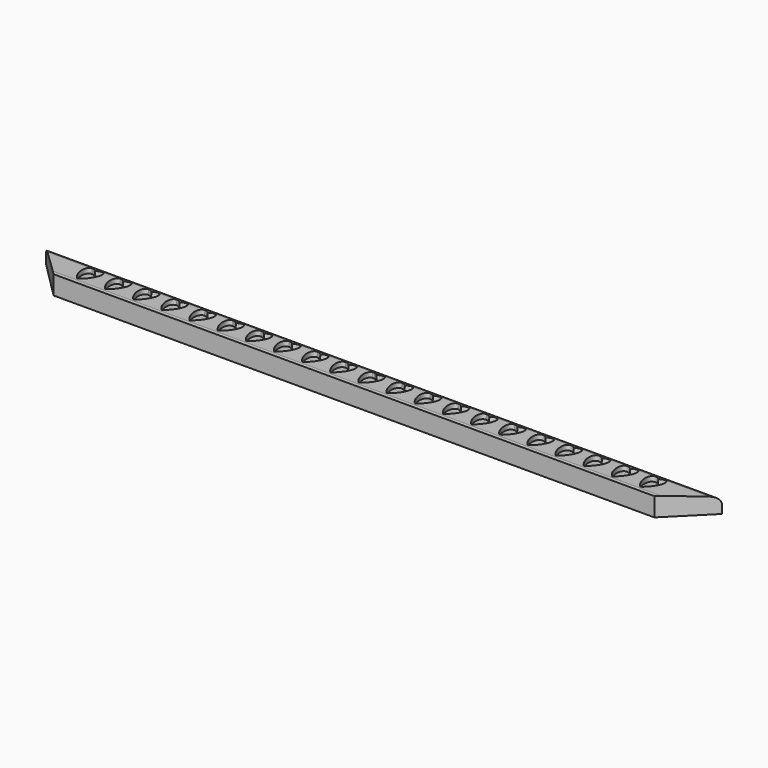
from build123d import *

# Parameters (mm, degrees)
F1_DEPTH = 12.7
F2_SIZE2 = 22.86
F2_SIZE  = 2.54
F3_R     = 5.08
F5_DEPTH = 3.175


# Not quite as in the source:
# - a feature names something its author has since deleted; it is built from what else it names


with BuildPart() as f1:
    # F0 (on Top) → F1 (new body)
    with BuildSketch(Plane.XY):
        Polygon((228.6, 12.7), (-228.6, 12.7), (-203.2, -12.7), (203.2, -12.7), align=None)
    extrude(amount=F1_DEPTH)

    # F2
    f2_edges = [f1.edges().sort_by_distance(p)[0] for p in [
        (0, 12.7, 12.7),
    ]]
    f2_side = f1.faces().sort_by_distance((0, 12.7, 6.35))[0]
    chamfer(f2_edges, length=F2_SIZE, length2=F2_SIZE2, reference=f2_side)

    # F3
    f3_edges = [f1.edges().sort_by_distance(p)[0] for p in [
        (0, 12.7, 10.16),
    ]]
    fillet(f3_edges, radius=F3_R)

    # F4 (on face) → F5 (cut)
    with BuildSketch(Plane(origin=(0, 1.27, 11.43), x_dir=(1, 0, 0), z_dir=(0, 0.1104315261, 0.9938837347))):
        with BuildLine():
            add(Edge.make_bspline(
                [(-190.5, 5.3298376858), (-192.2906218206, 6.9535217541), (-193.7692225246, 6.9535217364)],
                knots=[5.4853328791, 5.4853328791, 5.4853328791, 6.084603808, 6.084603808, 6.084603808], degree=2, weights=[1, 0.9554441533, 1]))
            add(Edge.make_bspline(
                [(-193.7692225246, 6.9535217364), (-209.2613622208, 6.95352155), (-190.5, -10.058738989)],
                knots=[6.084603808, 6.084603808, 6.084603808, 8.6269255327, 8.6269255327, 8.6269255327], degree=2, weights=[1, 0.2951719329, 1]))
            add(Edge.make_bspline(
                [(-190.5, -10.058738989), (-171.7386375737, 6.9535217364), (-187.2307775049, 6.9535217364)],
                knots=[3.9394450816, 3.9394450816, 3.9394450816, 6.4817668125, 6.4817668125, 6.4817668125], degree=2, weights=[1, 0.29517193, 1]))
            add(Edge.make_bspline(
                [(-187.2307775049, 6.9535217364), (-188.709378199, 6.9535217364), (-190.5, 5.3298376858)],
                knots=[0.1985815053, 0.1985815053, 0.1985815053, 0.797852428, 0.797852428, 0.797852428], degree=2, weights=[1, 0.9554441542, 1]))
        make_face()
        with BuildLine():
            add(Edge.make_bspline(
                [(-171.45, 5.3298376858), (-173.2406217996, 6.9535217351), (-174.719222493, 6.9535217364)],
                knots=[5.4853328791, 5.4853328791, 5.4853328791, 6.0846038014, 6.0846038014, 6.0846038014], degree=2, weights=[1, 0.9554441542, 1]))
            add(Edge.make_bspline(
                [(-174.719222493, 6.9535217364), (-190.2113624409, 6.9535217496), (-171.45, -10.058738989)],
                knots=[6.0846038014, 6.0846038014, 6.0846038014, 8.6269255327, 8.6269255327, 8.6269255327], degree=2, weights=[1, 0.2951719298, 1]))
            add(Edge.make_bspline(
                [(-171.45, -10.058738989), (-152.6886375737, 6.9535217364), (-168.1807775049, 6.9535217364)],
                knots=[3.9394450816, 3.9394450816, 3.9394450816, 6.4817668125, 6.4817668125, 6.4817668125], degree=2, weights=[1, 0.29517193, 1]))
            add(Edge.make_bspline(
                [(-168.1807775049, 6.9535217364), (-169.659378199, 6.9535217364), (-171.45, 5.3298376858)],
                knots=[0.1985815053, 0.1985815053, 0.1985815053, 0.797852428, 0.797852428, 0.797852428], degree=2, weights=[1, 0.9554441542, 1]))
        make_face()
        with BuildLine():
            add(Edge.make_bspline(
                [(-152.4, 5.3298376858), (-154.190621801, 6.9535217364), (-155.6692224951, 6.9535217364)],
                knots=[5.4853328791, 5.4853328791, 5.4853328791, 6.0846038019, 6.0846038019, 6.0846038019], degree=2, weights=[1, 0.9554441542, 1]))
            add(Edge.make_bspline(
                [(-155.6692224951, 6.9535217364), (-171.1613624263, 6.9535217363), (-152.4, -10.058738989)],
                knots=[6.0846038019, 6.0846038019, 6.0846038019, 8.6269255327, 8.6269255327, 8.6269255327], degree=2, weights=[1, 0.29517193, 1]))
            add(Edge.make_bspline(
                [(-152.4, -10.058738989), (-133.6386378713, 6.9535214665), (-149.1307774621, 6.9535217364)],
                knots=[3.9394450816, 3.9394450816, 3.9394450816, 6.4817668036, 6.4817668036, 6.4817668036], degree=2, weights=[1, 0.2951719342, 1]))
            add(Edge.make_bspline(
                [(-149.1307774621, 6.9535217364), (-150.6093781706, 6.9535217621), (-152.4, 5.3298376858)],
                knots=[0.1985814964, 0.1985814964, 0.1985814964, 0.797852428, 0.797852428, 0.797852428], degree=2, weights=[1, 0.9554441529, 1]))
        make_face()
        with BuildLine():
            add(Edge.make_bspline(
                [(-133.35, 5.3298376858), (-135.140621801, 6.9535217364), (-136.6192224951, 6.9535217364)],
                knots=[5.4853328791, 5.4853328791, 5.4853328791, 6.0846038019, 6.0846038019, 6.0846038019], degree=2, weights=[1, 0.9554441542, 1]))
            add(Edge.make_bspline(
                [(-136.6192224951, 6.9535217364), (-152.1113624263, 6.9535217363), (-133.35, -10.058738989)],
                knots=[6.0846038019, 6.0846038019, 6.0846038019, 8.6269255327, 8.6269255327, 8.6269255327], degree=2, weights=[1, 0.29517193, 1]))
            add(Edge.make_bspline(
                [(-133.35, -10.058738989), (-114.5886378713, 6.9535214665), (-130.0807774621, 6.9535217364)],
                knots=[3.9394450816, 3.9394450816, 3.9394450816, 6.4817668036, 6.4817668036, 6.4817668036], degree=2, weights=[1, 0.2951719342, 1]))
            add(Edge.make_bspline(
                [(-130.0807774621, 6.9535217364), (-131.5593781706, 6.9535217621), (-133.35, 5.3298376858)],
                knots=[0.1985814964, 0.1985814964, 0.1985814964, 0.797852428, 0.797852428, 0.797852428], degree=2, weights=[1, 0.9554441529, 1]))
        make_face()
        with BuildLine():
            add(Edge.make_bspline(
                [(-114.3, 5.3298376858), (-116.0906217421, 6.953521683), (-117.5692224063, 6.9535217364)],
                knots=[5.4853328791, 5.4853328791, 5.4853328791, 6.0846037833, 6.0846037833, 6.0846037833], degree=2, weights=[1, 0.9554441569, 1]))
            add(Edge.make_bspline(
                [(-117.5692224063, 6.9535217364), (-133.0613630431, 6.9535222957), (-114.3, -10.058738989)],
                knots=[6.0846037833, 6.0846037833, 6.0846037833, 8.6269255327, 8.6269255327, 8.6269255327], degree=2, weights=[1, 0.2951719211, 1]))
            add(Edge.make_bspline(
                [(-114.3, -10.058738989), (-95.5386373164, 6.9535219697), (-111.030777542, 6.9535217364)],
                knots=[3.9394450816, 3.9394450816, 3.9394450816, 6.4817668202, 6.4817668202, 6.4817668202], degree=2, weights=[1, 0.2951719263, 1]))
            add(Edge.make_bspline(
                [(-111.030777542, 6.9535217364), (-112.5093782236, 6.9535217141), (-114.3, 5.3298376858)],
                knots=[0.1985815131, 0.1985815131, 0.1985815131, 0.797852428, 0.797852428, 0.797852428], degree=2, weights=[1, 0.9554441553, 1]))
        make_face()
        with BuildLine():
            add(Edge.make_bspline(
                [(-95.25, -10.058738989), (-76.4886375737, 6.9535217364), (-91.9807775049, 6.9535217364)],
                knots=[3.9394450816, 3.9394450816, 3.9394450816, 6.4817668125, 6.4817668125, 6.4817668125], degree=2, weights=[1, 0.29517193, 1]))
            add(Edge.make_bspline(
                [(-91.9807775049, 6.9535217364), (-93.459378199, 6.9535217364), (-95.25, 5.3298376858)],
                knots=[0.1985815053, 0.1985815053, 0.1985815053, 0.797852428, 0.797852428, 0.797852428], degree=2, weights=[1, 0.9554441542, 1]))
            add(Edge.make_bspline(
                [(-95.25, 5.3298376858), (-97.0406217996, 6.9535217351), (-98.519222493, 6.9535217364)],
                knots=[5.4853328791, 5.4853328791, 5.4853328791, 6.0846038014, 6.0846038014, 6.0846038014], degree=2, weights=[1, 0.9554441542, 1]))
            add(Edge.make_bspline(
                [(-98.519222493, 6.9535217364), (-114.0113624409, 6.9535217496), (-95.25, -10.058738989)],
                knots=[6.0846038014, 6.0846038014, 6.0846038014, 8.6269255327, 8.6269255327, 8.6269255327], degree=2, weights=[1, 0.2951719298, 1]))
        make_face()
        with BuildLine():
            add(Edge.make_bspline(
                [(-76.2, -10.058738989), (-57.438637273, 6.953522009), (-72.9307775482, 6.9535217364)],
                knots=[3.9394450816, 3.9394450816, 3.9394450816, 6.4817668215, 6.4817668215, 6.4817668215], degree=2, weights=[1, 0.2951719256, 1]))
            add(Edge.make_bspline(
                [(-72.9307775482, 6.9535217364), (-74.4093782277, 6.9535217103), (-76.2, 5.3298376858)],
                knots=[0.1985815144, 0.1985815144, 0.1985815144, 0.797852428, 0.797852428, 0.797852428], degree=2, weights=[1, 0.9554441555, 1]))
            add(Edge.make_bspline(
                [(-76.2, 5.3298376858), (-77.9906218599, 6.9535217897), (-79.4692225838, 6.9535217364)],
                knots=[5.4853328791, 5.4853328791, 5.4853328791, 6.0846038204, 6.0846038204, 6.0846038204], degree=2, weights=[1, 0.9554441514, 1]))
            add(Edge.make_bspline(
                [(-79.4692225838, 6.9535217364), (-94.9613618094, 6.953521177), (-76.2, -10.058738989)],
                knots=[6.0846038204, 6.0846038204, 6.0846038204, 8.6269255327, 8.6269255327, 8.6269255327], degree=2, weights=[1, 0.2951719388, 1]))
        make_face()
        with BuildLine():
            add(Edge.make_bspline(
                [(-57.15, -10.058738989), (-38.3886375871, 6.9535217242), (-53.880777503, 6.9535217364)],
                knots=[3.9394450816, 3.9394450816, 3.9394450816, 6.4817668121, 6.4817668121, 6.4817668121], degree=2, weights=[1, 0.2951719302, 1]))
            add(Edge.make_bspline(
                [(-53.880777503, 6.9535217364), (-55.3593781977, 6.9535217375), (-57.15, 5.3298376858)],
                knots=[0.1985815049, 0.1985815049, 0.1985815049, 0.797852428, 0.797852428, 0.797852428], degree=2, weights=[1, 0.9554441541, 1]))
            add(Edge.make_bspline(
                [(-57.15, 5.3298376858), (-58.940621801, 6.9535217364), (-60.4192224951, 6.9535217364)],
                knots=[5.4853328791, 5.4853328791, 5.4853328791, 6.0846038019, 6.0846038019, 6.0846038019], degree=2, weights=[1, 0.9554441542, 1]))
            add(Edge.make_bspline(
                [(-60.4192224951, 6.9535217364), (-75.9113624263, 6.9535217363), (-57.15, -10.058738989)],
                knots=[6.0846038019, 6.0846038019, 6.0846038019, 8.6269255327, 8.6269255327, 8.6269255327], degree=2, weights=[1, 0.29517193, 1]))
        make_face()
        with BuildLine():
            add(Edge.make_bspline(
                [(-38.1, -10.058738989), (-19.3386369435, 6.9535223078), (-34.8307775956, 6.9535217364)],
                knots=[3.9394450816, 3.9394450816, 3.9394450816, 6.4817668315, 6.4817668315, 6.4817668315], degree=2, weights=[1, 0.2951719209, 1]))
            add(Edge.make_bspline(
                [(-34.8307775956, 6.9535217364), (-36.3093782592, 6.9535216818), (-38.1, 5.3298376858)],
                knots=[0.1985815243, 0.1985815243, 0.1985815243, 0.797852428, 0.797852428, 0.797852428], degree=2, weights=[1, 0.955444157, 1]))
            add(Edge.make_bspline(
                [(-38.1, 5.3298376858), (-39.890621801, 6.9535217364), (-41.3692224951, 6.9535217364)],
                knots=[5.4853328791, 5.4853328791, 5.4853328791, 6.0846038019, 6.0846038019, 6.0846038019], degree=2, weights=[1, 0.9554441542, 1]))
            add(Edge.make_bspline(
                [(-41.3692224951, 6.9535217364), (-56.8613624263, 6.9535217363), (-38.1, -10.058738989)],
                knots=[6.0846038019, 6.0846038019, 6.0846038019, 8.6269255327, 8.6269255327, 8.6269255327], degree=2, weights=[1, 0.29517193, 1]))
        make_face()
        with BuildLine():
            add(Edge.make_bspline(
                [(19.05, 5.3298376858), (17.2593782129, 6.9535217237), (15.7807775259, 6.9535217364)],
                knots=[5.4853328791, 5.4853328791, 5.4853328791, 6.0846037975, 6.0846037975, 6.0846037975], degree=2, weights=[1, 0.9554441548, 1]))
            add(Edge.make_bspline(
                [(15.7807775259, 6.9535217364), (0.2886374279, 6.9535218686), (19.05, -10.058738989)],
                knots=[6.0846037975, 6.0846037975, 6.0846037975, 8.6269255327, 8.6269255327, 8.6269255327], degree=2, weights=[1, 0.2951719279, 1]))
            add(Edge.make_bspline(
                [(19.05, -10.058738989), (37.8113620751, 6.9535214179), (22.3192225456, 6.9535217364)],
                knots=[3.9394450816, 3.9394450816, 3.9394450816, 6.4817668019, 6.4817668019, 6.4817668019], degree=2, weights=[1, 0.295171935, 1]))
            add(Edge.make_bspline(
                [(22.3192225456, 6.9535217364), (20.8406218345, 6.9535217667), (19.05, 5.3298376858)],
                knots=[0.1985814948, 0.1985814948, 0.1985814948, 0.797852428, 0.797852428, 0.797852428], degree=2, weights=[1, 0.9554441526, 1]))
        make_face()
        with BuildLine():
            add(Edge.make_bspline(
                [(38.1, 5.3298376858), (36.3093782153, 6.9535217216), (34.8307775295, 6.9535217364)],
                knots=[5.4853328791, 5.4853328791, 5.4853328791, 6.0846037967, 6.0846037967, 6.0846037967], degree=2, weights=[1, 0.9554441549, 1]))
            add(Edge.make_bspline(
                [(34.8307775295, 6.9535217364), (19.3386374032, 6.9535218909), (38.1, -10.058738989)],
                knots=[6.0846037967, 6.0846037967, 6.0846037967, 8.6269255327, 8.6269255327, 8.6269255327], degree=2, weights=[1, 0.2951719275, 1]))
            add(Edge.make_bspline(
                [(38.1, -10.058738989), (56.8613623982, 6.9535217109), (41.3692224991, 6.9535217364)],
                knots=[3.9394450816, 3.9394450816, 3.9394450816, 6.4817668117, 6.4817668117, 6.4817668117], degree=2, weights=[1, 0.2951719304, 1]))
            add(Edge.make_bspline(
                [(41.3692224991, 6.9535217364), (39.8906218037, 6.9535217388), (38.1, 5.3298376858)],
                knots=[0.1985815045, 0.1985815045, 0.1985815045, 0.797852428, 0.797852428, 0.797852428], degree=2, weights=[1, 0.9554441541, 1]))
        make_face()
        with BuildLine():
            add(Edge.make_bspline(
                [(57.15, 5.3298376858), (55.3593781853, 6.9535217488), (53.8807774843, 6.9535217364)],
                knots=[5.4853328791, 5.4853328791, 5.4853328791, 6.0846038062, 6.0846038062, 6.0846038062], degree=2, weights=[1, 0.9554441535, 1]))
            add(Edge.make_bspline(
                [(53.8807774843, 6.9535217364), (38.3886377172, 6.9535216063), (57.15, -10.058738989)],
                knots=[6.0846038062, 6.0846038062, 6.0846038062, 8.6269255327, 8.6269255327, 8.6269255327], degree=2, weights=[1, 0.295171932, 1]))
            add(Edge.make_bspline(
                [(57.15, -10.058738989), (75.9113621555, 6.9535214909), (60.419222534, 6.9535217364)],
                knots=[3.9394450816, 3.9394450816, 3.9394450816, 6.4817668044, 6.4817668044, 6.4817668044], degree=2, weights=[1, 0.2951719339, 1]))
            add(Edge.make_bspline(
                [(60.419222534, 6.9535217364), (58.9406218268, 6.9535217598), (57.15, 5.3298376858)],
                knots=[0.1985814972, 0.1985814972, 0.1985814972, 0.797852428, 0.797852428, 0.797852428], degree=2, weights=[1, 0.955444153, 1]))
        make_face()
        with BuildLine():
            add(Edge.make_bspline(
                [(171.45, -10.058738989), (190.2113625182, 6.9535218197), (174.7192224818, 6.9535217364)],
                knots=[3.9394450816, 3.9394450816, 3.9394450816, 6.4817668153, 6.4817668153, 6.4817668153], degree=2, weights=[1, 0.2951719286, 1]))
            add(Edge.make_bspline(
                [(174.7192224818, 6.9535217364), (173.2406217922, 6.9535217284), (171.45, 5.3298376858)],
                knots=[0.1985815081, 0.1985815081, 0.1985815081, 0.797852428, 0.797852428, 0.797852428], degree=2, weights=[1, 0.9554441546, 1]))
            add(Edge.make_bspline(
                [(171.45, 5.3298376858), (169.659378199, 6.9535217364), (168.1807775049, 6.9535217364)],
                knots=[5.4853328791, 5.4853328791, 5.4853328791, 6.0846038019, 6.0846038019, 6.0846038019], degree=2, weights=[1, 0.9554441542, 1]))
            add(Edge.make_bspline(
                [(168.1807775049, 6.9535217364), (152.6886375737, 6.9535217364), (171.45, -10.058738989)],
                knots=[6.0846038019, 6.0846038019, 6.0846038019, 8.6269255327, 8.6269255327, 8.6269255327], degree=2, weights=[1, 0.29517193, 1]))
        make_face()
        with BuildLine():
            add(Edge.make_bspline(
                [(152.4, -10.058738989), (171.1613625182, 6.9535218197), (155.6692224818, 6.9535217364)],
                knots=[3.9394450816, 3.9394450816, 3.9394450816, 6.4817668153, 6.4817668153, 6.4817668153], degree=2, weights=[1, 0.2951719286, 1]))
            add(Edge.make_bspline(
                [(155.6692224818, 6.9535217364), (154.1906217922, 6.9535217284), (152.4, 5.3298376858)],
                knots=[0.1985815081, 0.1985815081, 0.1985815081, 0.797852428, 0.797852428, 0.797852428], degree=2, weights=[1, 0.9554441546, 1]))
            add(Edge.make_bspline(
                [(152.4, 5.3298376858), (150.609378199, 6.9535217364), (149.1307775049, 6.9535217364)],
                knots=[5.4853328791, 5.4853328791, 5.4853328791, 6.0846038019, 6.0846038019, 6.0846038019], degree=2, weights=[1, 0.9554441542, 1]))
            add(Edge.make_bspline(
                [(149.1307775049, 6.9535217364), (133.6386375737, 6.9535217364), (152.4, -10.058738989)],
                knots=[6.0846038019, 6.0846038019, 6.0846038019, 8.6269255327, 8.6269255327, 8.6269255327], degree=2, weights=[1, 0.29517193, 1]))
        make_face()
        with BuildLine():
            add(Edge.make_bspline(
                [(133.35, -10.058738989), (152.1113625182, 6.9535218197), (136.6192224818, 6.9535217364)],
                knots=[3.9394450816, 3.9394450816, 3.9394450816, 6.4817668153, 6.4817668153, 6.4817668153], degree=2, weights=[1, 0.2951719286, 1]))
            add(Edge.make_bspline(
                [(136.6192224818, 6.9535217364), (135.1406217922, 6.9535217284), (133.35, 5.3298376858)],
                knots=[0.1985815081, 0.1985815081, 0.1985815081, 0.797852428, 0.797852428, 0.797852428], degree=2, weights=[1, 0.9554441546, 1]))
            add(Edge.make_bspline(
                [(133.35, 5.3298376858), (131.559378199, 6.9535217364), (130.0807775049, 6.9535217364)],
                knots=[5.4853328791, 5.4853328791, 5.4853328791, 6.0846038019, 6.0846038019, 6.0846038019], degree=2, weights=[1, 0.9554441542, 1]))
            add(Edge.make_bspline(
                [(130.0807775049, 6.9535217364), (114.5886375737, 6.9535217364), (133.35, -10.058738989)],
                knots=[6.0846038019, 6.0846038019, 6.0846038019, 8.6269255327, 8.6269255327, 8.6269255327], degree=2, weights=[1, 0.29517193, 1]))
        make_face()
        with BuildLine():
            add(Edge.make_bspline(
                [(114.3, -10.058738989), (133.0613625182, 6.9535218197), (117.5692224818, 6.9535217364)],
                knots=[3.9394450816, 3.9394450816, 3.9394450816, 6.4817668153, 6.4817668153, 6.4817668153], degree=2, weights=[1, 0.2951719286, 1]))
            add(Edge.make_bspline(
                [(117.5692224818, 6.9535217364), (116.0906217922, 6.9535217284), (114.3, 5.3298376858)],
                knots=[0.1985815081, 0.1985815081, 0.1985815081, 0.797852428, 0.797852428, 0.797852428], degree=2, weights=[1, 0.9554441546, 1]))
            add(Edge.make_bspline(
                [(114.3, 5.3298376858), (112.509378199, 6.9535217364), (111.0307775049, 6.9535217364)],
                knots=[5.4853328791, 5.4853328791, 5.4853328791, 6.0846038019, 6.0846038019, 6.0846038019], degree=2, weights=[1, 0.9554441542, 1]))
            add(Edge.make_bspline(
                [(111.0307775049, 6.9535217364), (95.5386375737, 6.9535217364), (114.3, -10.058738989)],
                knots=[6.0846038019, 6.0846038019, 6.0846038019, 8.6269255327, 8.6269255327, 8.6269255327], degree=2, weights=[1, 0.29517193, 1]))
        make_face()
        with BuildLine():
            add(Edge.make_bspline(
                [(95.25, 5.3298376858), (93.4593781644, 6.9535217677), (91.9807774528, 6.9535217364)],
                knots=[5.4853328791, 5.4853328791, 5.4853328791, 6.0846038128, 6.0846038128, 6.0846038128], degree=2, weights=[1, 0.9554441526, 1]))
            add(Edge.make_bspline(
                [(91.9807774528, 6.9535217364), (76.4886379361, 6.9535214077), (95.25, -10.058738989)],
                knots=[6.0846038128, 6.0846038128, 6.0846038128, 8.6269255327, 8.6269255327, 8.6269255327], degree=2, weights=[1, 0.2951719352, 1]))
            add(Edge.make_bspline(
                [(95.25, -10.058738989), (114.0113625182, 6.9535218197), (98.5192224818, 6.9535217364)],
                knots=[3.9394450816, 3.9394450816, 3.9394450816, 6.4817668153, 6.4817668153, 6.4817668153], degree=2, weights=[1, 0.2951719286, 1]))
            add(Edge.make_bspline(
                [(98.5192224818, 6.9535217364), (97.0406217922, 6.9535217284), (95.25, 5.3298376858)],
                knots=[0.1985815081, 0.1985815081, 0.1985815081, 0.797852428, 0.797852428, 0.797852428], degree=2, weights=[1, 0.9554441546, 1]))
        make_face()
        with BuildLine():
            add(Edge.make_bspline(
                [(76.2, 5.3298376858), (74.4093782111, 6.9535217254), (72.9307775232, 6.9535217364)],
                knots=[5.4853328791, 5.4853328791, 5.4853328791, 6.084603798, 6.084603798, 6.084603798], degree=2, weights=[1, 0.9554441547, 1]))
            add(Edge.make_bspline(
                [(72.9307775232, 6.9535217364), (57.4386374467, 6.9535218516), (76.2, -10.058738989)],
                knots=[6.084603798, 6.084603798, 6.084603798, 8.6269255327, 8.6269255327, 8.6269255327], degree=2, weights=[1, 0.2951719281, 1]))
            add(Edge.make_bspline(
                [(76.2, -10.058738989), (94.9613625182, 6.9535218197), (79.4692224818, 6.9535217364)],
                knots=[3.9394450816, 3.9394450816, 3.9394450816, 6.4817668153, 6.4817668153, 6.4817668153], degree=2, weights=[1, 0.2951719286, 1]))
            add(Edge.make_bspline(
                [(79.4692224818, 6.9535217364), (77.9906217922, 6.9535217284), (76.2, 5.3298376858)],
                knots=[0.1985815081, 0.1985815081, 0.1985815081, 0.797852428, 0.797852428, 0.797852428], degree=2, weights=[1, 0.9554441546, 1]))
        make_face()
        with BuildLine():
            Line((-2.5698701499, 6.8624797793), (-3.9046904667, 6.8624797793))
            add(Edge.make_bspline(
                [(-3.9046904667, 6.8624797793), (-14.9619228058, 3.5082997975), (0, -10.058738989)],
                knots=[6.2245075419, 6.2245075419, 6.2245075419, 8.6269255327, 8.6269255327, 8.6269255327], degree=2, weights=[1, 0.361230659, 1]))
            add(Edge.make_bspline(
                [(0, -10.058738989), (14.9619228058, 3.5082997975), (3.9046904667, 6.8624797793)],
                knots=[3.9394450816, 3.9394450816, 3.9394450816, 6.3418630724, 6.3418630724, 6.3418630724], degree=2, weights=[1, 0.361230659, 1]))
            Line((3.9046904667, 6.8624797793), (2.5698701499, 6.8624797793))
            add(Edge.make_bspline(
                [(2.5698701499, 6.8624797793), (1.3551785487, 6.5586743915), (0, 5.3298376858)],
                knots=[0.3384852454, 0.3384852454, 0.3384852454, 0.797852428, 0.797852428, 0.797852428], degree=2, weights=[1, 0.9737384803, 1]))
            add(Edge.make_bspline(
                [(0, 5.3298376858), (-1.3551785487, 6.5586743915), (-2.5698701499, 6.8624797793)],
                knots=[5.4853328791, 5.4853328791, 5.4853328791, 5.9447000618, 5.9447000618, 5.9447000618], degree=2, weights=[1, 0.9737384803, 1]))
        make_face()
        with BuildLine():
            add(Edge.make_bspline(
                [(-19.05, -10.058738989), (-0.2886376874, 6.9535216333), (-15.7807774886, 6.9535217364)],
                knots=[3.9394450816, 3.9394450816, 3.9394450816, 6.4817668091, 6.4817668091, 6.4817668091], degree=2, weights=[1, 0.2951719316, 1]))
            add(Edge.make_bspline(
                [(-15.7807774886, 6.9535217364), (-17.2593781882, 6.9535217462), (-19.05, 5.3298376858)],
                knots=[0.1985815019, 0.1985815019, 0.1985815019, 0.797852428, 0.797852428, 0.797852428], degree=2, weights=[1, 0.9554441537, 1]))
            add(Edge.make_bspline(
                [(-19.05, 5.3298376858), (-20.8406218144, 6.9535217485), (-22.3192225153, 6.9535217364)],
                knots=[5.4853328791, 5.4853328791, 5.4853328791, 6.0846038061, 6.0846038061, 6.0846038061], degree=2, weights=[1, 0.9554441536, 1]))
            add(Edge.make_bspline(
                [(-22.3192225153, 6.9535217364), (-37.8113622858, 6.953521609), (-19.05, -10.058738989)],
                knots=[6.0846038061, 6.0846038061, 6.0846038061, 8.6269255327, 8.6269255327, 8.6269255327], degree=2, weights=[1, 0.295171932, 1]))
        make_face()
        with BuildLine():
            add(Edge.make_bspline(
                [(190.5, -10.058738989), (209.2613625182, 6.9535218197), (193.7692224818, 6.9535217364)],
                knots=[3.9394450816, 3.9394450816, 3.9394450816, 6.4817668153, 6.4817668153, 6.4817668153], degree=2, weights=[1, 0.2951719286, 1]))
            add(Edge.make_bspline(
                [(193.7692224818, 6.9535217364), (192.2906217922, 6.9535217284), (190.5, 5.3298376858)],
                knots=[0.1985815081, 0.1985815081, 0.1985815081, 0.797852428, 0.797852428, 0.797852428], degree=2, weights=[1, 0.9554441546, 1]))
            add(Edge.make_bspline(
                [(190.5, 5.3298376858), (188.709378199, 6.9535217364), (187.2307775049, 6.9535217364)],
                knots=[5.4853328791, 5.4853328791, 5.4853328791, 6.0846038019, 6.0846038019, 6.0846038019], degree=2, weights=[1, 0.9554441542, 1]))
            add(Edge.make_bspline(
                [(187.2307775049, 6.9535217364), (171.7386375737, 6.9535217364), (190.5, -10.058738989)],
                knots=[6.0846038019, 6.0846038019, 6.0846038019, 8.6269255327, 8.6269255327, 8.6269255327], degree=2, weights=[1, 0.29517193, 1]))
        make_face()
    extrude(amount=-F5_DEPTH, mode=Mode.SUBTRACT)


solid = f1.part
